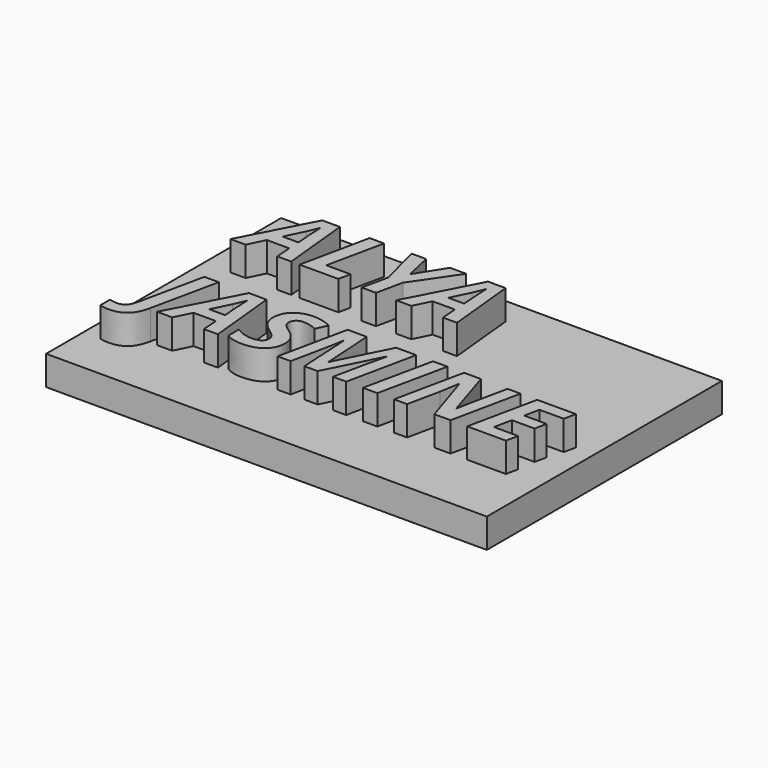
from build123d import *

# Parameters (mm, degrees)
F0_W         = 30
F0_H         = 20
F1_DEPTH     = 2
F2_TEXT_SIZE = 6.5963379004
F3_DEPTH     = 2


# Not quite as in the source:
# - Text() gives the source's letters only with a copy of the font that has no kerning and outlines rounded to 1/6400 em; it was checked with that copy


with BuildPart() as f1:
    # F0 (on Top) → F1 (new body)
    with BuildSketch(Plane.XY):
        with Locations((-9.969053655, 10)):
            Rectangle(F0_W, F0_H)
    extrude(amount=F1_DEPTH)

    # F2 (on face) → F3 (join)
    with BuildSketch(Plane.XY.offset(2)):
        with Locations((-22.7680663811, 13.4275276214)):
            Text('ALYA', F2_TEXT_SIZE, font='Open Sans', font_style=FontStyle.BOLDITALIC, text_align=(TextAlign.LEFT, TextAlign.BOTTOM))
        with Locations((-22.7680663811, 4.4565080769)):
            Text('JASMINE', F2_TEXT_SIZE, font='Open Sans', font_style=FontStyle.BOLDITALIC, text_align=(TextAlign.LEFT, TextAlign.BOTTOM))
    extrude(amount=F3_DEPTH)


solid = f1.part
